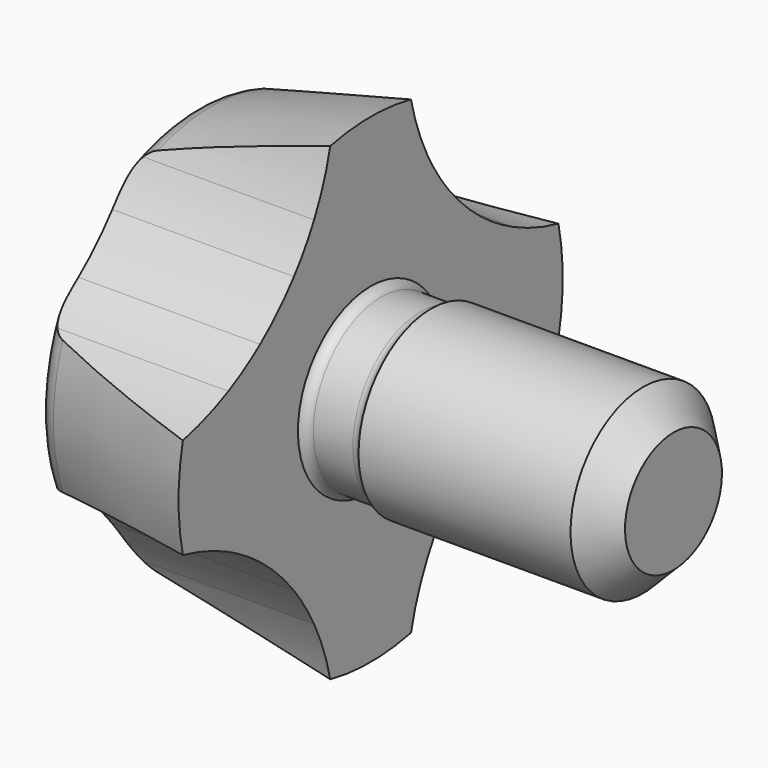
from build123d import *

# Parameters (mm, degrees)
F0_W     = 0.65359
F0_H     = 1.4
F0_W_2   = 3.5
F0_H_2   = 1.5
F3_DEPTH = 25


# Not quite as in the source:
# - ends of sketch curves that miss each other by under 0.0002 mm in the source are joined


with BuildPart() as f1:
    # F0 (on Front) → F1 (revolve)
    with BuildSketch(Plane.XZ):
        with BuildLine():
            ThreePointArc((9.366912, 1.4), (9.2669120175, 1.4267949091), (9.1937069394, 1.499999965))
            Line((9.193707, 1.499999965), (9.193707, 0))
            Line((9.193707, 0), (9.366912, 0))
            Line((9.366912, 0), (9.366912, 1.4))
        make_face()
        with Locations((9.693707, 0.7)):
            Rectangle(F0_W, F0_H)
        with BuildLine():
            ThreePointArc((10.1937070606, 1.499999965), (10.1205019825, 1.4267949091), (10.020502, 1.4))
            Line((10.020502, 1.4), (10.020502, 0))
            Line((10.020502, 0), (10.193707, 0))
            Line((10.193707, 0), (10.193707, 1.5))
        make_face()
        with Locations((11.943707, 0.75)):
            Rectangle(F0_W_2, F0_H_2)
        Polygon((14.193707, 1), (13.693707, 1.5), (13.693707, 0), (14.193707, 0), align=None)
        with BuildLine():
            Line((9.193707, 3.964102), (6.564298, 3.259553))
            ThreePointArc((6.5642979867, 3.2595530496), (6.2970304903, 3.0809709236), (6.193707, 2.77659))
            Line((6.193707, 2.77659), (6.193707, 0))
            Line((6.193707, 0), (9.193707, 0))
            Line((9.193707, 0), (9.193707, 1.499999965))
            Line((9.193707, 1.499999965), (9.193707, 3.964102))
        make_face()
    revolve(axis=Axis((10.368707, 0, 0), (-1, 0, 0)))

    # F2 (on face) → F3 (cut)
    with BuildSketch(Plane(origin=(6.193707, 0, 0), x_dir=(0, -1, 0), z_dir=(-1, 0, 0))):
        with BuildLine():
            ThreePointArc((3.8756311548, 0.8328191991), (2.8030435942, 2.8030432168), (0.8328197209, 3.8756310427))
            ThreePointArc((0.8328197209, 3.8756310427), (0.9707821759, 3.3957019848), (1.1674679485, 2.9367028921))
            ThreePointArc((1.1674679485, 2.9367028921), (1.3588439576, 2.5991932034), (1.5820188923, 2.2818124929))
            ThreePointArc((1.5820188923, 2.2818124929), (1.9633456176, 1.9633456176), (2.2818124929, 1.5820188923))
            ThreePointArc((2.2818124929, 1.5820188923), (2.599193614, 1.3588436976), (2.9367037599, 1.1674675107))
            ThreePointArc((2.9367037599, 1.1674675107), (3.3957025442, 0.9707819765), (3.8756311548, 0.8328191991))
        make_face()
        with BuildLine():
            ThreePointArc((-1.1674668381, 2.9367031109), (-0.9707811347, 3.3957021002), (-0.8328183948, 3.8756308663))
            ThreePointArc((-0.8328183948, 3.8756308663), (-2.8030431743, 2.8030436368), (-3.8756311107, 0.8328194045))
            ThreePointArc((-3.8756311107, 0.8328194045), (-3.3957018345, 0.970781873), (-2.9367033101, 1.167467233))
            ThreePointArc((-2.9367033101, 1.167467233), (-2.5991940372, 1.3588427967), (-2.281813665, 1.5820172017))
            ThreePointArc((-2.281813665, 1.5820172017), (-1.9633454104, 1.9633458247), (-1.5820167202, 2.2818139988))
            ThreePointArc((-1.5820167202, 2.2818139988), (-1.3588423817, 2.5991941131), (-1.1674668381, 2.9367031109))
        make_face()
        with BuildLine():
            ThreePointArc((2.2818124929, 1.5820188923), (1.9633456176, 1.9633456176), (1.5820188923, 2.2818124929))
            ThreePointArc((1.5820188923, 2.2818124929), (1.9101898753, 1.9101898753), (2.2818124929, 1.5820188923))
        make_face()
        with BuildLine():
            ThreePointArc((-2.281813665, 1.5820172017), (-1.9101891737, 1.9101895768), (-1.5820167202, 2.2818139988))
            ThreePointArc((-1.5820167202, 2.2818139988), (-1.9633454104, 1.9633458247), (-2.281813665, 1.5820172017))
        make_face()
        with BuildLine():
            ThreePointArc((-2.9367033101, -1.167467233), (-3.3957018345, -0.970781873), (-3.8756300769, -0.8328193482))
            ThreePointArc((-3.8756300769, -0.8328193482), (-2.8030431743, -2.8030436368), (-0.8328187651, -3.8756312481))
            ThreePointArc((-0.8328187651, -3.8756312481), (-0.9707811347, -3.3957021002), (-1.1674668381, -2.9367031109))
            ThreePointArc((-1.1674668381, -2.9367031109), (-1.3588423817, -2.5991941131), (-1.5820167202, -2.2818139988))
            ThreePointArc((-1.5820167202, -2.2818139988), (-1.9633454104, -1.9633458247), (-2.281813665, -1.5820172017))
            ThreePointArc((-2.281813665, -1.5820172017), (-2.5991940372, -1.3588427967), (-2.9367033101, -1.167467233))
        make_face()
        with BuildLine():
            ThreePointArc((0.8328197209, -3.8756310427), (2.8030435942, -2.8030432168), (3.8756311548, -0.8328191991))
            ThreePointArc((3.8756311548, -0.8328191991), (3.3957025442, -0.9707819765), (2.9367037599, -1.1674675107))
            ThreePointArc((2.9367037599, -1.1674675107), (2.599193614, -1.3588436976), (2.2818124929, -1.5820188923))
            ThreePointArc((2.2818124929, -1.5820188923), (1.9633456176, -1.9633456176), (1.5820188923, -2.2818124929))
            ThreePointArc((1.5820188923, -2.2818124929), (1.3588439576, -2.5991932034), (1.1674679485, -2.9367028921))
            ThreePointArc((1.1674679485, -2.9367028921), (0.9707821759, -3.3957019848), (0.8328197209, -3.8756310427))
        make_face()
        with BuildLine():
            ThreePointArc((1.5820188923, -2.2818124929), (1.9633456176, -1.9633456176), (2.2818124929, -1.5820188923))
            ThreePointArc((2.2818124929, -1.5820188923), (1.9101898753, -1.9101898753), (1.5820188923, -2.2818124929))
        make_face()
        with BuildLine():
            ThreePointArc((-1.5820167202, -2.2818139988), (-1.9101891737, -1.9101895768), (-2.281813665, -1.5820172017))
            ThreePointArc((-2.281813665, -1.5820172017), (-1.9633454104, -1.9633458247), (-1.5820167202, -2.2818139988))
        make_face()
    extrude(amount=-F3_DEPTH, mode=Mode.SUBTRACT)


solid = f1.part
